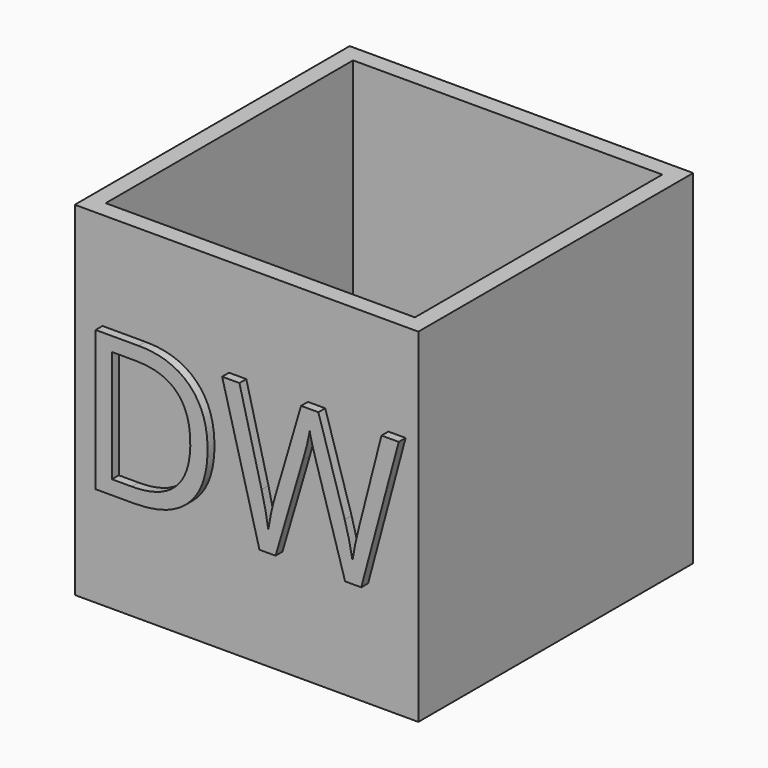
from build123d import *

# Parameters (mm, degrees)
F0_W         = 50.8
F0_H         = 50.8
F1_DEPTH     = 50.8
F2_T         = -2.54
F3_TEXT_SIZE = 29.0443241182
F4_DEPTH     = 1.27


# Not quite as in the source:
# - Text() gives the source's letters only with a copy of the font that has no kerning and outlines rounded to 1/6400 em; it was checked with that copy


with BuildPart() as f1:
    # F0 (on Front) → F1 (new body)
    with BuildSketch(Plane.XZ):
        with Locations((-46.2785235882, 52.1186686397)):
            Rectangle(F0_W, F0_H)
    extrude(amount=F1_DEPTH)

    # F2
    f2_openings = [f1.faces().sort_by_distance(p)[0] for p in [
        (-46.278524, -25.4, 77.518669),
    ]]
    offset(amount=F2_T, openings=f2_openings)

    # F3 (on face) → F4 (join)
    with BuildSketch(Plane.XZ.offset(50.8)):
        with Locations((-70.4308634393, 42.3358790576)):
            Text('DW', F3_TEXT_SIZE, font='Open Sans', text_align=(TextAlign.LEFT, TextAlign.BOTTOM))
    extrude(amount=F4_DEPTH)


solid = f1.part
